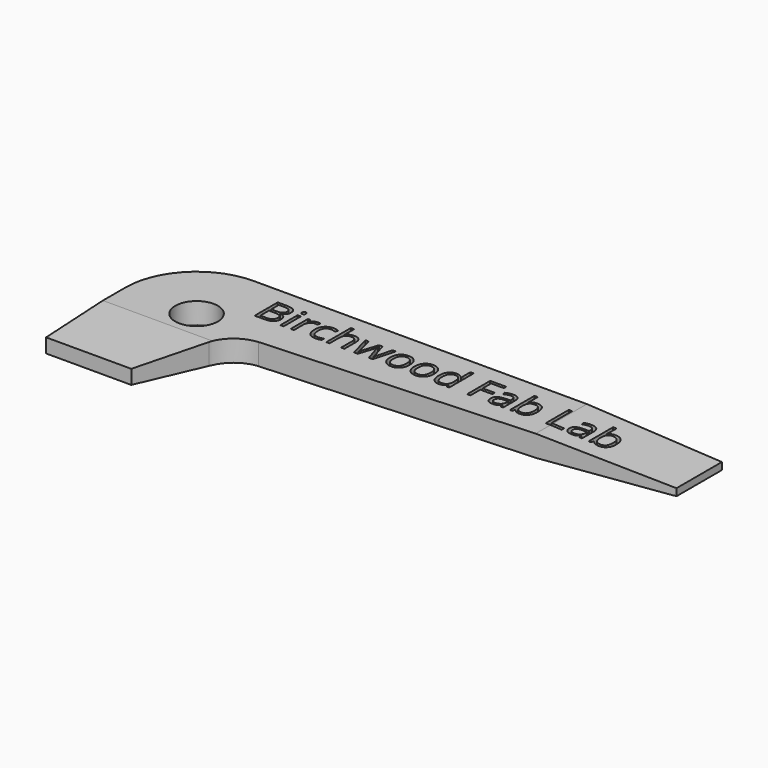
from build123d import *

# Parameters (mm, degrees)
F0_R          = 2.38125
F1_DEPTH      = 2.38125
F2_R          = 7.9375
F4_DEPTH      = 19.051
F6_DEPTH      = 9.5648146833
F8_DEPTH      = 19.051
F10_DEPTH     = 60.326
F11_TEXT_SIZE = 4.5180444979
F12_DEPTH     = 3.81


# Not quite as in the source:
# - Text() gives the source's letters only with a copy of the font that has no kerning and outlines rounded to 1/6400 em; it was checked with that copy


with BuildPart() as f1:
    # F0 (on Top) → F1 (new body)
    with BuildSketch(Plane.XY):
        with BuildLine():
            Line((6.8802531183, 46.4430405467), (-53.4447468817, 46.4430405467))
            Line((-53.4447468817, 46.4430405467), (-53.4447468817, 27.3930405467))
            Line((-53.4447468817, 27.3930405467), (-43.9197468817, 27.3930405467))
            Line((-43.9197468817, 27.3930405467), (-41.3273820942, 35.0202070092))
            ThreePointArc((-41.3273820942, 35.0202070092), (-40.0228140496, 36.8628863815), (-37.9243791103, 37.6959145069))
            Line((-37.9243791103, 37.6959145069), (6.8802531183, 40.0930405467))
            Line((6.8802531183, 40.0930405467), (6.8802531183, 46.4430405467))
        make_face()
        with Locations((-45.5072468817, 38.5055405467)):
            Circle(F0_R, mode=Mode.SUBTRACT)
    extrude(amount=F1_DEPTH)

    # F2
    f2_edges = [f1.edges().sort_by_distance(p)[0] for p in [
        (-53.444747, 46.443041, 1.190625),
    ]]
    fillet(f2_edges, radius=F2_R)

    # F3 (on face) → F4 (cut, through all)
    with BuildSketch(Plane(origin=(0, 46.4430405467, 0), x_dir=(-1, 0, 0), z_dir=(0, 1, 0))):
        Polygon((-7.2697603085, 1.5504802494), (-6.8802531183, 1.5907407505), (8.2211783156, 2.38125), (8.2030607001, 2.727358446), (-7.2193359956, 3.1990723219), align=None)
    extrude(amount=-F4_DEPTH, mode=Mode.SUBTRACT)

    # F5 (on face) → F6 (cut, through all)
    with BuildSketch(Plane(origin=(-2.1192870449, 39.6115494375, 0), x_dir=(0.9985718469, 0.053425337, 0), z_dir=(0.053425337, -0.9985718469, 0))):
        Polygon((9.0124112666, 0.7953703753), (-6.0780490749, 0), (9.0124112666, 0), align=None)
    extrude(amount=-F6_DEPTH, mode=Mode.SUBTRACT)

    # F7 (on face) → F8 (cut, through all)
    with BuildSketch(Plane(origin=(0, 46.4430405467, 0), x_dir=(-1, 0, 0), z_dir=(0, 1, 0))):
        Polygon((-6.5405170331, 0.7953703753), (-6.8802531183, 0.7953703753), (-6.9836541079, 0.7953703753), (-6.9836541079, -0.0977396412), (-6.5405170331, -0.0977396412), align=None)
    extrude(amount=-F8_DEPTH, mode=Mode.SUBTRACT)

    # F9 (on face) → F10 (cut, through all)
    with BuildSketch(Plane(origin=(-53.4447468817, 0, 0), x_dir=(0, -1, 0), z_dir=(-1, 0, 0))):
        Polygon((-35.3305405467, 2.38125), (-27.3930405467, 1.984375), (-26.6849351877, 1.984375), (-26.7145372927, 2.7254258748), align=None)
        Polygon((-26.9428193569, 0.396875), (-27.3930405467, 0.396875), (-35.3432405467, 0), (-35.0132025778, -0.3093605337), (-26.8219634891, -0.3093605337), align=None)
    extrude(amount=-F10_DEPTH, mode=Mode.SUBTRACT)

    # F11 (on face) → F12 (cut)
    with BuildSketch(Plane.XY.offset(2.38125)):
        with Locations((-41.7510472254, 41.3728742293)):
            Text('Birchwood Fab Lab', F11_TEXT_SIZE, font='Open Sans', text_align=(TextAlign.LEFT, TextAlign.BOTTOM))
    extrude(amount=-F12_DEPTH, mode=Mode.SUBTRACT)


solid = f1.part
